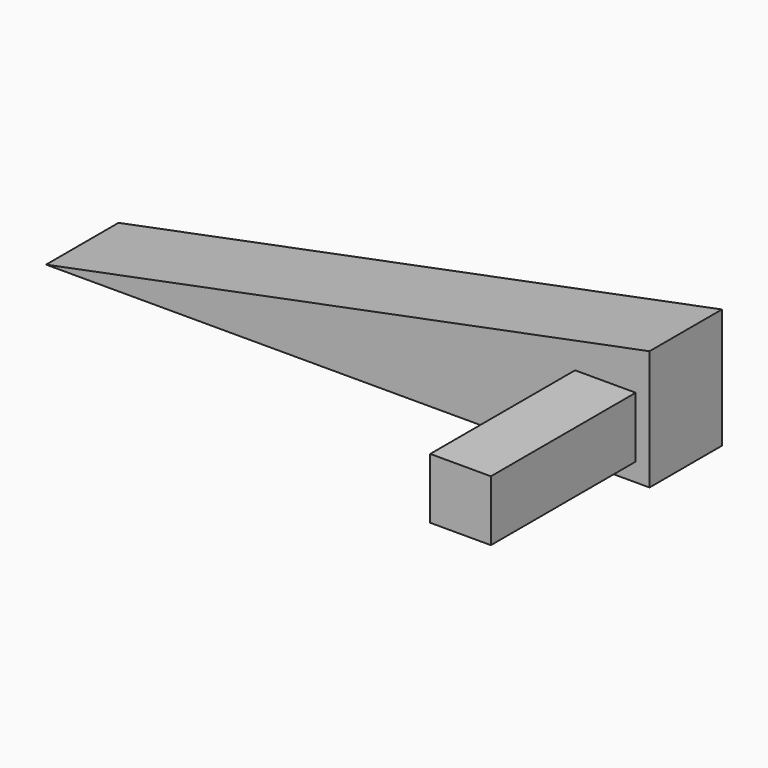
from build123d import *

# Parameters (mm, degrees)
F0_W        = 254
F0_H        = 50.8
F1_DEPTH    = 38.1
F2_T1_DEPTH = 1365.7843192567
F3_W        = 25.5302116275
F3_H        = 25.5302092992
F4_DEPTH    = 76.2


# Not quite as in the source:
# - a fillet or chamfer that OpenCascade refuses, or shapes differently, is made with other operations: its cross-section is extruded or revolved along the edge and cut away or added


with BuildPart() as f1:
    # F0 (on Front) → F1 (new body)
    with BuildSketch(Plane.XZ):
        with Locations((-22.1173410591, 25.4)):
            Rectangle(F0_W, F0_H)
    extrude(amount=F1_DEPTH)

    # F2: chamfer of 50.8 x 255.5053741775 on 1 edges, made by hand

    # F2_s2 → F2_t1 (cut)
    with BuildSketch(Plane.XZ.offset(-663.8421596283)):
        Polygon((106.3880331184, 50.8), (-149.1173410591, 0), (-149.1173410591, 50.8), align=None)
    extrude(amount=F2_T1_DEPTH, mode=Mode.SUBTRACT)

    # F3 (on face) → F4 (join)
    with BuildSketch(Plane.XZ.offset(38.1)):
        with Locations((86.3100104034, 20.4800155479)):
            Rectangle(F3_W, F3_H)
    extrude(amount=F4_DEPTH)


solid = f1.part
